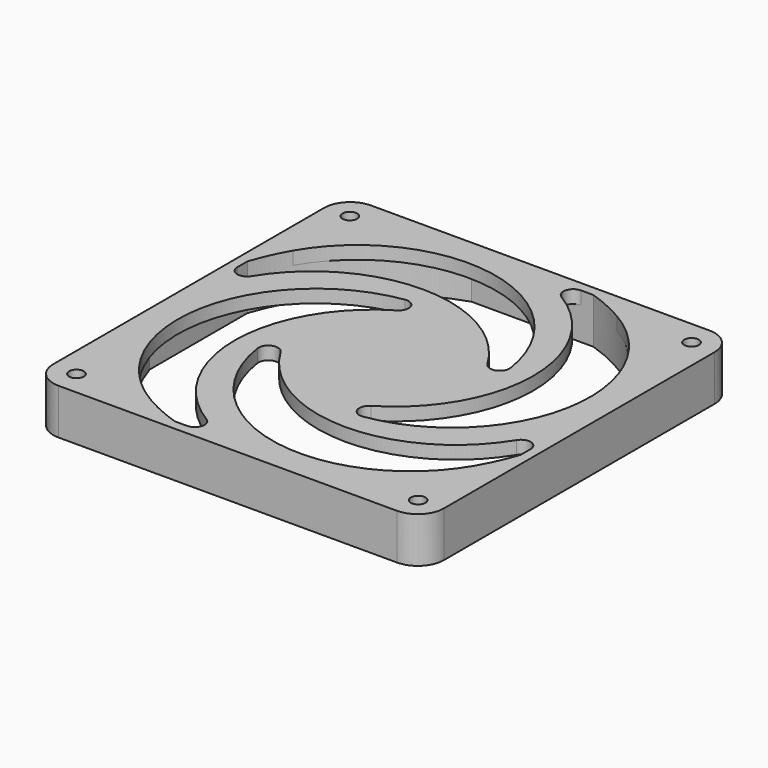
from build123d import *

# Parameters (mm, degrees)
F0_R            = 25
F0_R_2          = 2.25
F1_DEPTH        = 14
F2_DEPTH        = 10
F4_DEPTH        = 14.001
F5_R            = 3
F7_DEPTH        = 12
F7_COPIES_COUNT = 4


# Not quite as in the source:
# - a pattern or mirror of a feature is missing from the dataset's text; its kind, count and spacing are read off the source's solid


with BuildPart() as f1:
    # F0 (on Top) → F1 (new body)
    with BuildSketch(Plane.XY):
        with BuildLine():
            ThreePointArc((57, 18.7349939952), (42.4264068712, 42.4264068712), (18.7349939952, 57))
            Line((18.7349939952, 57), (-18.7349939952, 57))
            ThreePointArc((-18.7349939952, 57), (-42.4264068712, 42.4264068712), (-57, 18.7349939952))
            Line((-57, 18.7349939952), (-57, -18.7349939952))
            ThreePointArc((-57, -18.7349939952), (-42.4264068712, -42.4264068712), (-18.7349939952, -57))
            Line((-18.7349939952, -57), (18.7349939952, -57))
            ThreePointArc((18.7349939952, -57), (42.4264068712, -42.4264068712), (57, -18.7349939952))
            Line((57, -18.7349939952), (57, 18.7349939952))
        make_face()
        Circle(F0_R, mode=Mode.SUBTRACT)
        Circle(F0_R)
        with BuildLine():
            ThreePointArc((-18.7349939952, 57), (-9.486832838, 59.2452529972), (2.885e-07, 60))
            Line((2.885e-07, 60), (-52, 60))
            ThreePointArc((-52, 60), (-57.6568542495, 57.6568542495), (-60, 52))
            Line((-60, 52), (-60, 2.895e-07))
            ThreePointArc((-60, 2.895e-07), (-59.2452529515, 9.4868331234), (-57, 18.7349939952))
            ThreePointArc((-57, 18.7349939952), (-42.4264068712, 42.4264068712), (-18.7349939952, 57))
        make_face()
        with Locations((-52.5, 52.5)):
            Circle(F0_R_2, mode=Mode.SUBTRACT)
        with BuildLine():
            ThreePointArc((-57, -18.7349939952), (-59.2452529973, -9.4868328376), (-60, 2.895e-07))
            Line((-60, 2.895e-07), (-60, -52))
            ThreePointArc((-60, -52), (-57.6568542495, -57.6568542495), (-52, -60))
            Line((-52, -60), (-2.57e-07, -60))
            ThreePointArc((-2.57e-07, -60), (-9.4868331074, -59.2452529541), (-18.7349939952, -57))
            ThreePointArc((-18.7349939952, -57), (-42.4264068712, -42.4264068712), (-57, -18.7349939952))
        make_face()
        with Locations((-52.5, -52.5)):
            Circle(F0_R_2, mode=Mode.SUBTRACT)
        with BuildLine():
            Line((60, -52), (60, 0))
            ThreePointArc((60, 0), (59.2452529744, -9.4868329805), (57, -18.7349939952))
            ThreePointArc((57, -18.7349939952), (42.4264068712, -42.4264068712), (18.7349939952, -57))
            ThreePointArc((18.7349939952, -57), (9.4868328536, -59.2452529947), (-2.57e-07, -60))
            Line((-2.57e-07, -60), (52, -60))
            ThreePointArc((52, -60), (57.6568542495, -57.6568542495), (60, -52))
        make_face()
        with Locations((52.5, -52.5)):
            Circle(F0_R_2, mode=Mode.SUBTRACT)
        with BuildLine():
            ThreePointArc((60, 52), (57.6568542495, 57.6568542495), (52, 60))
            Line((52, 60), (2.885e-07, 60))
            ThreePointArc((2.885e-07, 60), (9.486833123, 59.2452529516), (18.7349939952, 57))
            ThreePointArc((18.7349939952, 57), (42.4264068712, 42.4264068712), (57, 18.7349939952))
            ThreePointArc((57, 18.7349939952), (59.2452529744, 9.4868329805), (60, 0))
            Line((60, 0), (60, 52))
        make_face()
        with Locations((52.5, 52.5)):
            Circle(F0_R_2, mode=Mode.SUBTRACT)
        with BuildLine():
            ThreePointArc((18.7349939952, 57), (9.486833123, 59.2452529516), (2.885e-07, 60))
            ThreePointArc((2.885e-07, 60), (-9.486832838, 59.2452529972), (-18.7349939952, 57))
            Line((-18.7349939952, 57), (18.7349939952, 57))
        make_face()
        with BuildLine():
            Line((-57, -18.7349939952), (-57, 18.7349939952))
            ThreePointArc((-57, 18.7349939952), (-59.2452529515, 9.4868331234), (-60, 2.895e-07))
            ThreePointArc((-60, 2.895e-07), (-59.2452529973, -9.4868328376), (-57, -18.7349939952))
        make_face()
        with BuildLine():
            ThreePointArc((-2.57e-07, -60), (9.4868328536, -59.2452529947), (18.7349939952, -57))
            Line((18.7349939952, -57), (-18.7349939952, -57))
            ThreePointArc((-18.7349939952, -57), (-9.4868331074, -59.2452529541), (-2.57e-07, -60))
        make_face()
        with BuildLine():
            ThreePointArc((57, -18.7349939952), (59.2452529744, -9.4868329805), (60, 0))
            ThreePointArc((60, 0), (59.2452529744, 9.4868329805), (57, 18.7349939952))
            Line((57, 18.7349939952), (57, -18.7349939952))
        make_face()
    extrude(amount=F1_DEPTH)

    # F0 (on Top) → F2 (cut)
    with BuildSketch(Plane.XY):
        with BuildLine():
            ThreePointArc((57, 18.7349939952), (42.4264068712, 42.4264068712), (18.7349939952, 57))
            Line((18.7349939952, 57), (-18.7349939952, 57))
            ThreePointArc((-18.7349939952, 57), (-42.4264068712, 42.4264068712), (-57, 18.7349939952))
            Line((-57, 18.7349939952), (-57, -18.7349939952))
            ThreePointArc((-57, -18.7349939952), (-42.4264068712, -42.4264068712), (-18.7349939952, -57))
            Line((-18.7349939952, -57), (18.7349939952, -57))
            ThreePointArc((18.7349939952, -57), (42.4264068712, -42.4264068712), (57, -18.7349939952))
            Line((57, -18.7349939952), (57, 18.7349939952))
        make_face()
        Circle(F0_R, mode=Mode.SUBTRACT)
        Circle(F0_R)
    extrude(amount=F2_DEPTH, mode=Mode.SUBTRACT)

    # F3 (on face) → F4 (cut, through all)
    with BuildSketch(Plane.XY):
        with BuildLine():
            ThreePointArc((51.9615242271, -30), (54.7711468799, -24.4973767873), (57, -18.7349939952))
            Line((57, -18.7349939952), (57, 1.314733996))
            ThreePointArc((57, 1.314733996), (22.5078780664, -33.1091892137), (-21.6506350946, -12.5))
            ThreePointArc((-21.6506350946, -12.5), (-25, 0), (-21.6506350946, 12.5))
            ThreePointArc((-21.6506350946, 12.5), (-6.0945554338, -45.5560796608), (51.9615242271, -30))
        make_face()
        with BuildLine():
            Line((-18.7349939952, -57), (1.314733996, -57))
            ThreePointArc((1.314733996, -57), (-33.1091892137, -22.5078780664), (-12.5, 21.6506350946))
            ThreePointArc((-12.5, 21.6506350946), (0, 25), (12.5, 21.6506350946))
            ThreePointArc((12.5, 21.6506350946), (-45.5560796608, 6.0945554338), (-30, -51.9615242271))
            ThreePointArc((-30, -51.9615242271), (-24.4973767873, -54.7711468799), (-18.7349939952, -57))
        make_face()
        with BuildLine():
            ThreePointArc((-12.5, -21.6506350946), (45.5560796608, -6.0945554338), (30, 51.9615242271))
            ThreePointArc((30, 51.9615242271), (24.4973767873, 54.7711468799), (18.7349939952, 57))
            Line((18.7349939952, 57), (-1.314733996, 57))
            ThreePointArc((-1.314733996, 57), (33.1091892137, 22.5078780664), (12.5, -21.6506350946))
            ThreePointArc((12.5, -21.6506350946), (0, -25), (-12.5, -21.6506350946))
        make_face()
        with BuildLine():
            ThreePointArc((25, 0), (24.1481456572, -6.4704761276), (21.6506350946, -12.5))
            ThreePointArc((21.6506350946, -12.5), (6.0945554338, 45.5560796608), (-51.9615242271, 30))
            ThreePointArc((-51.9615242271, 30), (-54.7711468799, 24.4973767873), (-57, 18.7349939952))
            Line((-57, 18.7349939952), (-57, -1.314733996))
            ThreePointArc((-57, -1.314733996), (-22.5078780664, 33.1091892137), (21.6506350946, 12.5))
            ThreePointArc((21.6506350946, 12.5), (24.1481456572, 6.4704761276), (25, 0))
        make_face()
    extrude(amount=F4_DEPTH, mode=Mode.SUBTRACT)

    # F5
    f5_edges = [f1.edges().sort_by_distance(p)[0] for p in [
        (21.650635, -12.5, 12),
        (12.5, 21.650635, 12),
        (-21.650635, 12.5, 12),
        (-12.5, -21.650635, 12),
        (-57, -1.314734, 12),
        (-1.314734, 57, 12),
        (57, 1.314734, 12),
        (1.314734, -57, 12),
    ]]
    fillet(f5_edges, radius=F5_R)

    # F6 (on face) → F7 (cut)
    with BuildSketch(Plane.XY):
        with BuildLine():
            ThreePointArc((58, -21.9089023002), (43.8406204336, -43.8406204336), (21.9089023002, -58))
            Line((21.9089023002, -58), (48.1010791024, -58))
            ThreePointArc((48.1010791024, -58), (49.0271170017, -57.3774305355), (48.8001090628, -56.2849076182))
            ThreePointArc((48.8001090628, -56.2849076182), (48.7573593129, -48.7573593129), (56.2849076182, -48.8001090628))
            ThreePointArc((56.2849076182, -48.8001090628), (57.3774305355, -49.0271170017), (58, -48.1010791024))
            Line((58, -48.1010791024), (58, -21.9089023002))
        make_face()
    f7 = extrude(amount=F7_DEPTH, mode=Mode.SUBTRACT)

    # F7_copies: F7 ×4 about axis
    f7_copies_axis = Axis((0, 0, 0), (0, 0, 1))
    for i in range(1, F7_COPIES_COUNT):
        add(f7.rotate(f7_copies_axis, i * 360 / F7_COPIES_COUNT), mode=Mode.SUBTRACT)


solid = f1.part
